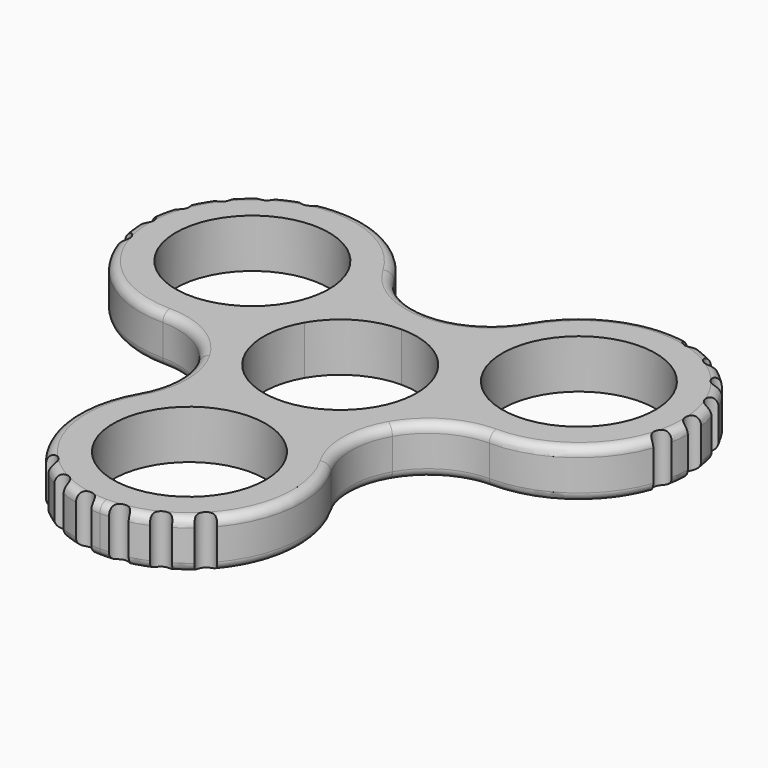
from build123d import *

# Parameters (mm, degrees)
F0_R     = 10.9363137741
F1_DEPTH = 7.00024
F3_DEPTH = 7.00124
F5_R     = 1.27


# Not quite as in the source:
# - a feature of the source that left no trace in its solid (it failed there, or was rolled back) is left out


with BuildPart() as f1:
    # F0 (on Top) → F1 (new body)
    with BuildSketch(Plane.XY):
        with BuildLine():
            ThreePointArc((0, 10.99058), (5.49529, 9.5181214823), (9.5181214823, 5.49529))
            Line((9.5181214823, 5.49529), (13.9175305336, 8.03529))
            ThreePointArc((13.9175305336, 8.03529), (17.9403620159, 23.0487014823), (32.9537734982, 19.02587))
            Line((32.9537734982, 19.02587), (37.3531825494, 21.56587))
            ThreePointArc((37.3531825494, 21.56587), (23.4356520159, 29.60116), (9.5181214823, 21.56587))
            ThreePointArc((9.5181214823, 21.56587), (5.49529, 17.5430385177), (0, 16.07058))
            Line((0, 16.07058), (0, 10.99058))
        make_face()
        with BuildLine():
            Line((13.9175305336, 8.03529), (9.5181214823, 5.49529))
            ThreePointArc((9.5181214823, 5.49529), (10.99058, 0), (9.5181214823, -5.49529))
            Line((9.5181214823, -5.49529), (13.9175305336, -8.03529))
            ThreePointArc((13.9175305336, -8.03529), (17.9403620159, -4.0124585177), (23.4356520159, -2.54))
            ThreePointArc((23.4356520159, -2.54), (37.3531825494, 5.49529), (37.3531825494, 21.56587))
            Line((37.3531825494, 21.56587), (32.9537734982, 19.02587))
            ThreePointArc((32.9537734982, 19.02587), (28.9309420159, 4.0124585177), (13.9175305336, 8.03529))
        make_face()
        with BuildLine():
            Line((13.9175305336, -8.03529), (9.5181214823, -5.49529))
            ThreePointArc((9.5181214823, -5.49529), (0, -10.99058), (-9.5181214823, -5.49529))
            Line((-9.5181214823, -5.49529), (-13.9175305336, -8.03529))
            ThreePointArc((-13.9175305336, -8.03529), (-12.4450720159, -13.53058), (-13.9175305336, -19.02587))
            ThreePointArc((-13.9175305336, -19.02587), (-13.9175305336, -35.09645), (0, -43.13174))
            ThreePointArc((0, -43.13174), (13.9175305336, -35.09645), (13.9175305336, -19.02587))
            ThreePointArc((13.9175305336, -19.02587), (12.4450720159, -13.53058), (13.9175305336, -8.03529))
        make_face()
        with Locations((0, -27.06116)):
            Circle(F0_R, mode=Mode.SUBTRACT)
        with BuildLine():
            ThreePointArc((-9.5181214823, 5.49529), (-5.49529, 9.5181214823), (0, 10.99058))
            Line((0, 10.99058), (0, 16.07058))
            ThreePointArc((0, 16.07058), (-5.49529, 17.5430385177), (-9.5181214823, 21.56587))
            ThreePointArc((-9.5181214823, 21.56587), (-23.4356520159, 29.60116), (-37.3531825494, 21.56587))
            Line((-37.3531825494, 21.56587), (-32.9537734982, 19.02587))
            ThreePointArc((-32.9537734982, 19.02587), (-17.9403620159, 23.0487014823), (-13.9175305336, 8.03529))
            Line((-13.9175305336, 8.03529), (-9.5181214823, 5.49529))
        make_face()
        with BuildLine():
            Line((-13.9175305336, -8.03529), (-9.5181214823, -5.49529))
            ThreePointArc((-9.5181214823, -5.49529), (-10.99058, 0), (-9.5181214823, 5.49529))
            Line((-9.5181214823, 5.49529), (-13.9175305336, 8.03529))
            ThreePointArc((-13.9175305336, 8.03529), (-28.9309420159, 4.0124585177), (-32.9537734982, 19.02587))
            Line((-32.9537734982, 19.02587), (-37.3531825494, 21.56587))
            ThreePointArc((-37.3531825494, 21.56587), (-37.3531825494, 5.49529), (-23.4356520159, -2.54))
            ThreePointArc((-23.4356520159, -2.54), (-17.9403620159, -4.0124585177), (-13.9175305336, -8.03529))
        make_face()
    extrude(amount=F1_DEPTH)

    # F2 (on face) → F3 (cut, through all)
    with BuildSketch(Plane.XY.offset(7.00024)):
        with BuildLine():
            ThreePointArc((-35.0746224958, 24.6120017365), (-35.9139467032, 23.6575589786), (-36.6752197739, 22.6397724514))
            ThreePointArc((-36.6752197739, 22.6397724514), (-34.8888064923, 22.8255884549), (-35.0746224958, 24.6120017365))
        make_face()
        with BuildLine():
            ThreePointArc((-37.9442279658, 20.4417857879), (-38.4450204186, 19.2736107058), (-38.8519299897, 18.0695132413))
            ThreePointArc((-38.8519299897, 18.0695132413), (-37.2119427044, 18.8017985026), (-37.9442279658, 20.4417857879))
        make_face()
        with BuildLine():
            ThreePointArc((-39.3814291193, 15.5295132413), (-39.4895877236, 14.2618048815), (-39.4971210738, 12.9895132413))
            ThreePointArc((-39.4971210738, 12.9895132413), (-38.1692750966, 14.201667264), (-39.3814291193, 15.5295132413))
        make_face()
        with BuildLine():
            ThreePointArc((-31.0484267333, 27.6836433659), (-32.1430835358, 27.0377698581), (-33.1832757705, 26.3074095236))
            ThreePointArc((-33.1832757705, 26.3074095236), (-31.4277343308, 25.9281019262), (-31.0484267333, 27.6836433659))
        make_face()
        with BuildLine():
            ThreePointArc((-39.2112581719, 10.4656506457), (-38.9197100236, 9.2285468584), (-38.5313098328, 8.0183520828))
            ThreePointArc((-38.5313098328, 8.0183520828), (-37.6476347209, 9.5819755338), (-39.2112581719, 10.4656506457))
        make_face()
        with BuildLine():
            ThreePointArc((-26.2662923178, 29.3499041644), (-27.507583715, 29.0767343082), (-28.7234053742, 28.7063240001))
            ThreePointArc((-28.7234053742, 28.7063240001), (-27.1730587639, 27.799557554), (-26.2662923178, 29.3499041644))
        make_face()
        with BuildLine():
            ThreePointArc((26.2662923178, 29.3499041644), (27.1730587639, 27.799557554), (28.7234053742, 28.7063240001))
            ThreePointArc((28.7234053742, 28.7063240001), (27.507583715, 29.0767343082), (26.2662923178, 29.3499041644))
        make_face()
        with BuildLine():
            ThreePointArc((31.0484267333, 27.6836433659), (31.4277343308, 25.9281019262), (33.1832757705, 26.3074095236))
            ThreePointArc((33.1832757705, 26.3074095236), (32.1430835358, 27.0377698581), (31.0484267333, 27.6836433659))
        make_face()
        with BuildLine():
            ThreePointArc((35.0746224958, 24.6120017365), (34.8888064923, 22.8255884549), (36.6752197739, 22.6397724514))
            ThreePointArc((36.6752197739, 22.6397724514), (35.9139467032, 23.6575589786), (35.0746224958, 24.6120017365))
        make_face()
        with BuildLine():
            ThreePointArc((37.9442279658, 20.4417857879), (37.2119427044, 18.8017985026), (38.8519299897, 18.0695132413))
            ThreePointArc((38.8519299897, 18.0695132413), (38.4450204186, 19.2736107058), (37.9442279658, 20.4417857879))
        make_face()
        with BuildLine():
            ThreePointArc((39.3814291193, 15.5295132413), (38.1692750966, 14.201667264), (39.4971210738, 12.9895132413))
            ThreePointArc((39.4971210738, 12.9895132413), (39.4895877236, 14.2618048815), (39.3814291193, 15.5295132413))
        make_face()
        with BuildLine():
            ThreePointArc((39.2112581719, 10.4656506457), (37.6476347209, 9.5819755338), (38.5313098328, 8.0183520828))
            ThreePointArc((38.5313098328, 8.0183520828), (38.9197100236, 9.2285468584), (39.2112581719, 10.4656506457))
        make_face()
        with BuildLine():
            ThreePointArc((1.2690081918, -43.0815582393), (2.5310737154, -42.9311696844), (3.7773074939, -42.6815149778))
            ThreePointArc((3.7773074939, -42.6815149778), (2.3231362121, -41.6273869575), (1.2690081918, -43.0815582393))
        make_face()
        with BuildLine():
            ThreePointArc((6.19124707, -41.8912645598), (7.3438537909, -41.355611827), (8.4505250575, -40.7305479815))
            ThreePointArc((8.4505250575, -40.7305479815), (6.7405277746, -40.1812672769), (6.19124707, -41.8912645598))
        make_face()
        with BuildLine():
            ThreePointArc((10.4987031463, -39.2283607373), (11.4273987125, -38.360633448), (12.2846164461, -37.4222284926))
            ThreePointArc((12.2846164461, -37.4222284926), (10.4885936738, -37.432337965), (10.4987031463, -39.2283607373))
        make_face()
        with BuildLine():
            ThreePointArc((-3.7773074939, -42.6815149778), (-2.5310737154, -42.9311696844), (-1.2690081918, -43.0815582393))
            ThreePointArc((-1.2690081918, -43.0815582393), (-2.3231362121, -41.6273869575), (-3.7773074939, -42.6815149778))
        make_face()
        with BuildLine():
            ThreePointArc((-8.4505250575, -40.7305479815), (-7.3438537909, -41.355611827), (-6.19124707, -41.8912645598))
            ThreePointArc((-6.19124707, -41.8912645598), (-6.7405277746, -40.1812672769), (-8.4505250575, -40.7305479815))
        make_face()
        with BuildLine():
            ThreePointArc((-12.2846164461, -37.4222284926), (-11.4273987125, -38.360633448), (-10.4987031463, -39.2283607373))
            ThreePointArc((-10.4987031463, -39.2283607373), (-10.4885936738, -37.432337965), (-12.2846164461, -37.4222284926))
        make_face()
    extrude(amount=-F3_DEPTH, mode=Mode.SUBTRACT)

    # F5
    f5_edges = [f1.edges().sort_by_distance(p)[0] for p in [
        (29.906152, 28.24099, 0),
        (34.162497, 25.497131, 0),
        (37.353183, 21.56587, 0),
        (39.168024, 16.810217, 0),
        (39.404131, 11.721925, 0),
        (39.404131, 11.721925, 7.00024),
        (39.168024, 16.810217, 7.00024),
        (37.353183, 21.56587, 7.00024),
        (34.162497, 25.497131, 7.00024),
        (29.906152, 28.24099, 7.00024),
        (-39.404131, 11.721925, 0),
        (-39.168024, 16.810217, 0),
        (-37.353183, 21.56587, 0),
        (-34.162497, 25.497131, 0),
        (-29.906152, 28.24099, 0),
        (-29.906152, 28.24099, 7.00024),
        (-34.162497, 25.497131, 7.00024),
        (-37.353183, 21.56587, 7.00024),
        (-39.168024, 16.810217, 7.00024),
        (-39.404131, 11.721925, 7.00024),
        (-9.504339, -40.019983, 7.00024),
        (-4.999914, -42.334156, 7.00024),
        (0, -43.13174, 7.00024),
        (4.999914, -42.334156, 7.00024),
        (9.504339, -40.019983, 7.00024),
        (9.504339, -40.019983, 0),
        (4.999914, -42.334156, 0),
        (0, -43.13174, 0),
        (-4.999914, -42.334156, 0),
        (-9.504339, -40.019983, 0),
        (16.662353, 28.104048, 0),
        (32.646484, 0.361521, 0),
        (13.917531, -8.03529, 0),
        (16.007643, -28.482045, 0),
        (-16.007643, -28.482045, 0),
        (-13.917531, -8.03529, 0),
        (-32.646484, 0.361521, 0),
        (-16.662353, 28.104048, 0),
        (0, 16.07058, 0),
        (16.662353, 28.104048, 7.00024),
        (32.646484, 0.361521, 7.00024),
        (13.917531, -8.03529, 7.00024),
        (16.007643, -28.482045, 7.00024),
        (-16.007643, -28.482045, 7.00024),
        (-13.917531, -8.03529, 7.00024),
        (-32.646484, 0.361521, 7.00024),
        (-16.662353, 28.104048, 7.00024),
        (0, 16.07058, 7.00024),
    ]]
    fillet(f5_edges, radius=F5_R)


solid = f1.part
